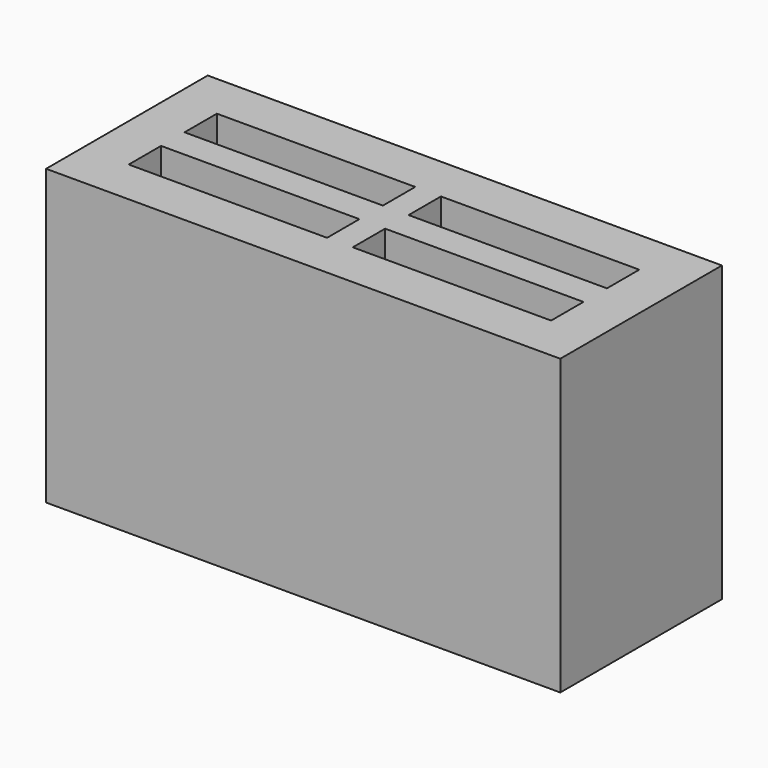
from build123d import *

# Parameters (mm, degrees)
F0_W     = 280
F0_H     = 110
F1_DEPTH = 160
F2_T     = -10
F3_W     = 260
F3_H     = 90
F3_W_2   = 108
F3_H_2   = 16
F3_W_3   = 14
F4_DEPTH = 150
F5_DEPTH = 40
F6_R     = 9
F7_DEPTH = 25


with BuildPart() as f1:
    # F0 (on Top) → F1 (new body)
    with BuildSketch(Plane.XY):
        Rectangle(F0_W, F0_H)
    extrude(amount=F1_DEPTH)

    # F2
    f2_openings = [f1.faces().sort_by_distance(p)[0] for p in [
        (0, 0, 160),
    ]]
    offset(amount=F2_T, openings=f2_openings)

    # F3 (on face) → F4 (join)
    with BuildSketch(Plane.XY.offset(10)):
        Rectangle(F3_W, F3_H)
        Polygon((115, 30), (115, 24.33777228), (115, 8), (115, -8), (115, -26.8225744367), (115, -30), (7, -30), (-7, -30), (-115, -30), (-115, -8), (-115, 8), (-115, 30), (-15, 30), (-7, 30), (7, 30), align=None, mode=Mode.SUBTRACT)
        with Locations((61, 0)):
            Rectangle(F3_W_2, F3_H_2)
        Polygon((-7, -8), (-7, 8), (-109.6588596702, 8), (-115, 8), (-115, -8), (-109.6588596702, -8), align=None)
        Polygon((-7, 8), (7, 8), (7, 30), (-7, 30), (-7, 15.2422059327), align=None)
        Polygon((7, -16.3514893502), (7, -8), (-7, -8), (-7, -30), (7, -30), align=None)
        Rectangle(F3_W_3, F3_H_2)
    extrude(amount=F4_DEPTH)

    # F3 (on face) → F5 (join)
    with BuildSketch(Plane.XY.offset(10)):
        Rectangle(F3_W, F3_H)
        Polygon((115, 30), (115, 24.33777228), (115, 8), (115, -8), (115, -26.8225744367), (115, -30), (7, -30), (-7, -30), (-115, -30), (-115, -8), (-115, 8), (-115, 30), (-15, 30), (-7, 30), (7, 30), align=None, mode=Mode.SUBTRACT)
        Polygon((115, 8), (115, 24.33777228), (115, 30), (7, 30), (7, 8), align=None)
        Polygon((115, -26.8225744367), (115, -8), (7, -8), (7, -16.3514893502), (7, -30), (115, -30), align=None)
        Polygon((-109.6588596702, 8), (-7, 8), (-7, 15.2422059327), (-7, 30), (-15, 30), (-115, 30), (-115, 8), align=None)
        Polygon((-7, -30), (-7, -8), (-109.6588596702, -8), (-115, -8), (-115, -30), align=None)
        with Locations((61, 0)):
            Rectangle(F3_W_2, F3_H_2)
        Polygon((-7, -8), (-7, 8), (-109.6588596702, 8), (-115, 8), (-115, -8), (-109.6588596702, -8), align=None)
        Rectangle(F3_W_3, F3_H_2)
    extrude(amount=F5_DEPTH)

    # F6 (on face) → F7 (cut)
    with BuildSketch(Plane(origin=(-140, 0, 0), x_dir=(0, -1, 0), z_dir=(-1, 0, 0))):
        with Locations((0, 25.6529357284)):
            Circle(F6_R)
    extrude(amount=-F7_DEPTH, mode=Mode.SUBTRACT)


solid = f1.part
